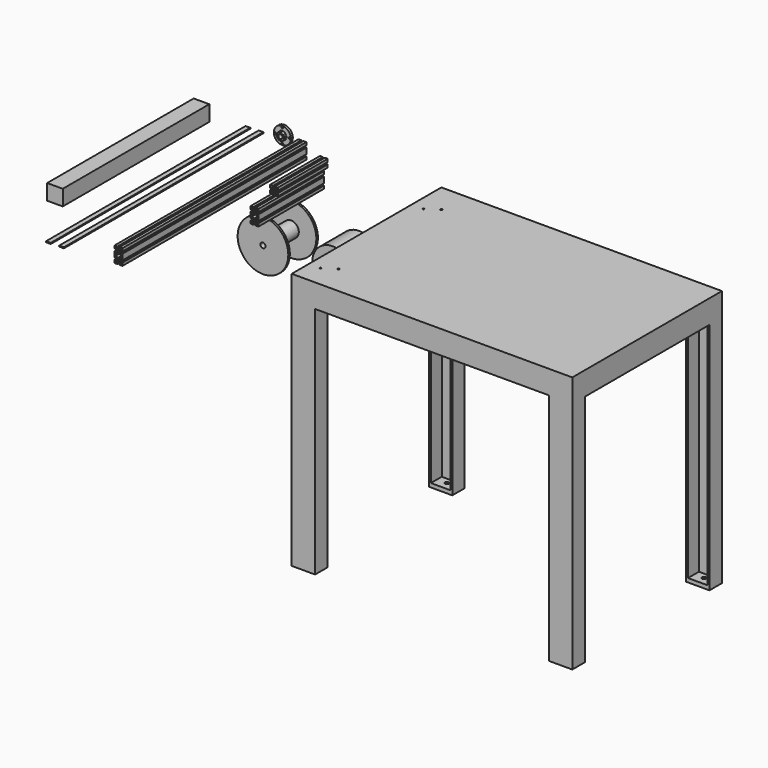
from build123d import *

# Parameters (mm, degrees)
F0_R      = 2.6035
F1_DEPTH  = 749.3
F2_R      = 2.6035
F3_DEPTH  = 203.2
F4_R      = 27.78125
F5_DEPTH  = 7.9375
F6_R      = 12.7
F6_R_2    = 6.858
F7_DEPTH  = 7.9375
F8_R      = 1.27
F10_DEPTH = 76.2
F12_DEPTH = 762
F13_R     = 82.55
F13_R_2   = 8.255
F14_DEPTH = 6.35
F15_R     = 25.4
F15_R_2   = 8.255
F16_DEPTH = 107.95
F17_R     = 82.55
F17_R_2   = 25.4
F17_R_3   = 8.255
F18_DEPTH = 6.35
F19_R     = 66.675
F19_R_2   = 8.255
F20_DEPTH = 107.95
F21_R     = 2.6035
F22_DEPTH = 266.7
F23_W     = 15.24
F23_H     = 3.175
F24_DEPTH = 812.8
F25_W     = 15.24
F25_H     = 3.175
F26_DEPTH = 812.8
F28_DEPTH = 12.7
F30_DEPTH = 12.7
F32_DEPTH = 12.7
F34_DEPTH = 12.7
F35_W     = 50.8
F35_H     = 596.9
F36_DEPTH = 50.8


with BuildPart() as f1:
    # F0 (on Front) → F1 (new body)
    with BuildSketch(Plane.XZ):
        Polygon((-3.2385, 4.5085), (-4.5085, 4.5085), (-4.5085, 3.2385), (-4.5085, -3.2385), (-4.5085, -4.5085), (-3.2385, -4.5085), (3.2385, -4.5085), (4.5085, -4.5085), (4.5085, -3.2385), (4.5085, 3.2385), (4.5085, 4.5085), (3.2385, 4.5085), align=None)
        Circle(F0_R, mode=Mode.SUBTRACT)
        Polygon((-4.5085, -4.5085), (-4.5085, -3.2385), (-10.4902, -7.4295), (-10.4902, -3.2385), (-12.7, -3.2385), (-12.7, -12.7), (-3.2385, -12.7), (-3.2385, -10.4902), (-7.4295, -10.4902), (-3.2385, -4.5085), align=None)
        Polygon((10.4902, -7.4295), (4.5085, -3.2385), (4.5085, -4.5085), (3.2385, -4.5085), (7.4295, -10.4902), (3.2385, -10.4902), (3.2385, -12.7), (12.7, -12.7), (12.7, -3.2385), (10.4902, -3.2385), align=None)
        Polygon((-4.5085, 3.2385), (-4.5085, 4.5085), (-3.2385, 4.5085), (-7.4295, 10.4902), (-7.432806, 12.7), (-12.7, 12.7), (-12.7, 3.2385), (-10.4902, 3.2385), (-10.4902, 7.4295), align=None)
        Polygon((-12.7, 12.7), (-7.432806, 12.7), (-7.436155, 14.938361), (-3.265166, 20.8915), (-4.5085, 20.8915), (-4.5085, 22.1615), (-10.4902, 17.999061), (-10.4902, 22.1615), (-12.7, 22.1615), align=None)
        Polygon((7.4295, 10.4902), (3.2385, 4.5085), (4.5085, 4.5085), (4.5085, 3.2385), (10.4902, 7.4295), (10.4902, 3.2385), (12.7, 3.2385), (12.7, 12.7), (7.426194, 12.7), align=None)
        Polygon((-12.7, 38.1), (-12.7, 28.6385), (-10.4902, 28.6385), (-10.4902, 32.858061), (-4.5085, 28.6385), (-4.5085, 29.9085), (-3.2385, 29.9085), (-7.436155, 35.8902), (-3.2385, 35.8902), (-3.2385, 38.1), align=None)
        Polygon((-4.5085, 20.8915), (-3.265166, 20.8915), (3.251856, 20.8915), (4.5085, 20.8915), (4.5085, 22.1615), (4.5085, 28.6385), (4.5085, 29.9085), (3.2385, 29.9085), (0, 29.9085), (-3.2385, 29.9085), (-4.5085, 29.9085), (-4.5085, 28.6385), (-4.5085, 22.1615), align=None)
        with BuildLine():
            ThreePointArc((2.6035, 25.4), (-1.840953, 23.559047), (0, 28.0035))
            ThreePointArc((0, 28.0035), (1.840953, 27.240953), (2.6035, 25.4))
        make_face(mode=Mode.SUBTRACT)
        Polygon((10.4902, 28.6385), (12.7, 28.6385), (12.7, 38.1), (3.2385, 38.1), (3.2385, 35.8902), (7.422845, 35.8902), (3.2385, 29.9085), (4.5085, 29.9085), (4.5085, 28.6385), (10.4902, 32.858061), align=None)
        Polygon((7.422845, 14.938361), (7.426194, 12.7), (12.7, 12.7), (12.7, 22.1615), (10.4902, 22.1615), (10.4902, 17.999061), (4.5085, 22.1615), (4.5085, 20.8915), (3.251856, 20.8915), align=None)
    extrude(amount=F1_DEPTH)


with BuildPart() as f3:
    # F2 (on Front) → F3 (new body)
    with BuildSketch(Plane.XZ):
        Polygon((65.21165, -4.37637), (65.21165, -3.10637), (59.22995, -7.29737), (59.22995, -3.10637), (57.02015, -3.10637), (57.02015, -12.56787), (66.48165, -12.56787), (66.48165, -10.35807), (62.29065, -10.35807), (66.48165, -4.37637), align=None)
        Polygon((65.21165, 3.37063), (65.21165, 4.64063), (66.48165, 4.64063), (62.29065, 10.62233), (66.48165, 10.62233), (66.48165, 12.83213), (57.02015, 12.83213), (57.02015, 3.37063), (59.22995, 3.37063), (59.22995, 7.56163), align=None)
        Polygon((77.14965, 10.62233), (72.95865, 4.64063), (74.22865, 4.64063), (74.22865, 3.37063), (80.21035, 7.56163), (80.21035, 4.291052), (80.21035, 3.37063), (82.42015, 3.37063), (82.42015, 12.83213), (72.95865, 12.83213), (72.95865, 10.62233), align=None)
        Polygon((80.21035, -7.29737), (74.22865, -3.10637), (74.22865, -4.37637), (72.95865, -4.37637), (77.14965, -10.35807), (72.95865, -10.35807), (72.95865, -12.56787), (82.42015, -12.56787), (82.42015, -3.10637), (80.21035, -3.10637), align=None)
        Polygon((66.48165, 4.64063), (65.21165, 4.64063), (65.21165, 3.37063), (65.21165, -3.10637), (65.21165, -4.37637), (66.48165, -4.37637), (72.95865, -4.37637), (74.22865, -4.37637), (74.22865, -3.10637), (74.22865, 3.37063), (74.22865, 4.64063), (72.95865, 4.64063), align=None)
        with Locations((69.72015, 0.13213)):
            Circle(F2_R, mode=Mode.SUBTRACT)
    extrude(amount=F3_DEPTH)


with BuildPart() as f5:
    # F4 (on Front) → F5 (new body)
    with BuildSketch(Plane.XZ):
        with Locations((-59.230567, 36.74075)):
            Circle(F4_R)
        with BuildLine():
            ThreePointArc((-56.062631, 60.341583), (-42.392587, 53.57873), (-35.629734, 39.908687))
            ThreePointArc((-35.629734, 39.908687), (-33.249129, 39.059442), (-32.243067, 36.74075))
            ThreePointArc((-32.243067, 36.74075), (-33.249129, 34.422058), (-35.629734, 33.572813))
            ThreePointArc((-35.629734, 33.572813), (-42.392587, 19.90277), (-56.062631, 13.139917))
            ThreePointArc((-56.062631, 13.139917), (-56.057333, 13.034142), (-56.055567, 12.92825))
            ThreePointArc((-56.055567, 12.92825), (-59.336459, 9.755016), (-62.398504, 13.139917))
            ThreePointArc((-62.398504, 13.139917), (-76.068547, 19.90277), (-82.8314, 33.572813))
            ThreePointArc((-82.8314, 33.572813), (-86.218067, 36.74075), (-82.8314, 39.908687))
            ThreePointArc((-82.8314, 39.908687), (-76.068547, 53.57873), (-62.398504, 60.341583))
            ThreePointArc((-62.398504, 60.341583), (-59.336459, 63.726484), (-56.055567, 60.55325))
            ThreePointArc((-56.055567, 60.55325), (-56.057333, 60.447358), (-56.062631, 60.341583))
        make_face(mode=Mode.SUBTRACT)
        with BuildLine():
            Line((-59.230567, 43.59875), (-59.230567, 57.37825))
            ThreePointArc((-59.230567, 57.37825), (-61.399505, 58.234558), (-62.398504, 60.341583))
            ThreePointArc((-62.398504, 60.341583), (-76.068547, 53.57873), (-82.8314, 39.908687))
            ThreePointArc((-82.8314, 39.908687), (-80.724375, 38.909688), (-79.868067, 36.74075))
            Line((-79.868067, 36.74075), (-66.088567, 36.74075))
            ThreePointArc((-66.088567, 36.74075), (-64.079905, 41.590088), (-59.230567, 43.59875))
        make_face()
        with BuildLine():
            ThreePointArc((-35.629734, 33.572813), (-38.593067, 36.74075), (-35.629734, 39.908687))
            ThreePointArc((-35.629734, 39.908687), (-42.392587, 53.57873), (-56.062631, 60.341583))
            ThreePointArc((-56.062631, 60.341583), (-57.061629, 58.234558), (-59.230567, 57.37825))
            Line((-59.230567, 57.37825), (-59.230567, 43.59875))
            ThreePointArc((-59.230567, 43.59875), (-54.381229, 41.590088), (-52.372567, 36.74075))
            ThreePointArc((-52.372567, 36.74075), (-59.230567, 29.88275), (-66.088567, 36.74075))
            Line((-66.088567, 36.74075), (-79.868067, 36.74075))
            ThreePointArc((-79.868067, 36.74075), (-80.724375, 34.571812), (-82.8314, 33.572813))
            ThreePointArc((-82.8314, 33.572813), (-76.068547, 19.90277), (-62.398504, 13.139917))
            ThreePointArc((-62.398504, 13.139917), (-59.230567, 16.10325), (-56.062631, 13.139917))
            ThreePointArc((-56.062631, 13.139917), (-42.392587, 19.90277), (-35.629734, 33.572813))
        make_face()
    extrude(amount=F5_DEPTH)

    # F6 (on face) → F7 (join)
    with BuildSketch(Plane.XZ.offset(7.9375)):
        with Locations((-59.230567, 36.74075)):
            Circle(F6_R)
        with Locations((-59.230567, 36.74075)):
            Circle(F6_R_2, mode=Mode.SUBTRACT)
    extrude(amount=F7_DEPTH)

    # F8
    f8_edges = [f5.edges().sort_by_distance(p)[0] for p in [
        (-71.930567, -15.875, 36.74075),
        (-71.930567, -7.9375, 36.74075),
    ]]
    fillet(f8_edges, radius=F8_R)


with BuildPart() as f10:
    # F9 (on Top) → F10 (new body)
    with BuildSketch(Plane.XY):
        Polygon((520.913526, -37.587471), (482.813526, -37.587471), (482.813526, -647.187471), (1397.213526, -647.187471), (1397.213526, -37.587471), (559.013526, -37.587471), align=None)
        with BuildLine():
            ThreePointArc((520.913526, -580.115596), (518.135401, -577.337471), (520.913526, -574.559346))
            ThreePointArc((520.913526, -574.559346), (522.877957, -575.37304), (523.691651, -577.337471))
            ThreePointArc((523.691651, -577.337471), (522.877957, -579.301902), (520.913526, -580.115596))
        make_face(mode=Mode.SUBTRACT)
        with BuildLine():
            ThreePointArc((559.013526, -555.112471), (555.838526, -551.937471), (559.013526, -548.762471))
            ThreePointArc((559.013526, -548.762471), (561.25859, -549.692407), (562.188526, -551.937471))
            ThreePointArc((562.188526, -551.937471), (561.25859, -554.182535), (559.013526, -555.112471))
        make_face(mode=Mode.SUBTRACT)
        with BuildLine():
            ThreePointArc((520.913526, -161.015596), (518.135401, -158.237471), (520.913526, -155.459346))
            ThreePointArc((520.913526, -155.459346), (522.877957, -156.27304), (523.691651, -158.237471))
            ThreePointArc((523.691651, -158.237471), (522.877957, -160.201902), (520.913526, -161.015596))
        make_face(mode=Mode.SUBTRACT)
        with BuildLine():
            ThreePointArc((559.013526, -136.012471), (555.838526, -132.837471), (559.013526, -129.662471))
            ThreePointArc((559.013526, -129.662471), (561.25859, -130.592407), (562.188526, -132.837471))
            ThreePointArc((562.188526, -132.837471), (561.25859, -135.082535), (559.013526, -136.012471))
        make_face(mode=Mode.SUBTRACT)
    extrude(amount=F10_DEPTH)

    # F11 (on face) → F12 (join)
    with BuildSketch(Plane(origin=(0, 0, 0), x_dir=(1, 0, 0), z_dir=(0, 0, -1))):
        Polygon((559.013526, 647.187471), (482.813526, 647.187471), (482.813526, 596.387471), (489.163518, 596.387471), (489.163518, 640.83748), (552.663534, 640.83748), (552.663534, 596.387471), (559.013526, 596.387471), align=None)
        Polygon((489.163526, 88.387471), (482.813526, 88.387471), (482.813526, 37.587471), (559.013526, 37.587471), (559.013526, 88.387471), (552.663526, 88.387471), (552.663526, 43.937471), (489.163526, 43.937471), align=None)
        Polygon((1397.213526, 647.187471), (1321.013526, 647.187471), (1321.013526, 596.387471), (1327.363558, 596.387471), (1327.363558, 640.837439), (1390.863494, 640.837439), (1390.863494, 596.387471), (1397.213526, 596.387471), align=None)
        Polygon((1397.213526, 37.587471), (1397.213526, 88.387471), (1390.863526, 88.387471), (1390.863526, 43.937471), (1327.363526, 43.937471), (1327.363526, 88.387471), (1321.013526, 88.387471), (1321.013526, 37.587471), align=None)
    extrude(amount=F12_DEPTH)

    # F27 (on face) → F28 (join)
    with BuildSketch(Plane(origin=(0, 0, -762), x_dir=(1, 0, 0), z_dir=(0, 0, -1))):
        with BuildLine():
            Line((549.488538, 640.83748), (492.338514, 640.83748))
            Line((492.338514, 640.83748), (515.630007, 625.309818))
            ThreePointArc((515.630007, 625.309818), (520.913526, 628.137471), (526.197046, 625.309818))
            Line((526.197046, 625.309818), (549.488538, 640.83748))
        make_face()
        with BuildLine():
            Line((515.630007, 625.309818), (492.338514, 640.83748))
            Line((492.338514, 640.83748), (489.163518, 640.83748))
            Line((489.163518, 640.83748), (489.163518, 600.620799))
            Line((489.163518, 600.620799), (515.630007, 618.265125))
            ThreePointArc((515.630007, 618.265125), (514.563526, 621.787471), (515.630007, 625.309818))
        make_face()
        with BuildLine():
            Line((489.163518, 600.620799), (489.163518, 596.387471))
            Line((489.163518, 596.387471), (552.663534, 596.387471))
            Line((552.663534, 596.387471), (552.663534, 600.620799))
            Line((552.663534, 600.620799), (526.197046, 618.265125))
            ThreePointArc((526.197046, 618.265125), (520.913526, 615.437471), (515.630007, 618.265125))
            Line((515.630007, 618.265125), (489.163518, 600.620799))
        make_face()
        with BuildLine():
            Line((552.663534, 640.83748), (549.488538, 640.83748))
            Line((549.488538, 640.83748), (526.197046, 625.309818))
            ThreePointArc((526.197046, 625.309818), (526.991061, 623.627601), (527.263526, 621.787471))
            ThreePointArc((527.263526, 621.787471), (526.991061, 619.947342), (526.197046, 618.265125))
            Line((526.197046, 618.265125), (552.663534, 600.620799))
            Line((552.663534, 600.620799), (552.663534, 640.83748))
        make_face()
    extrude(amount=-F28_DEPTH)

    # F29 (on face) → F30 (join)
    with BuildSketch(Plane(origin=(0, 0, -762), x_dir=(1, 0, 0), z_dir=(0, 0, -1))):
        with BuildLine():
            Line((552.663526, 88.387471), (489.163526, 88.387471))
            Line((489.163526, 88.387471), (489.163526, 84.154138))
            Line((489.163526, 84.154138), (515.630007, 66.509818))
            ThreePointArc((515.630007, 66.509818), (520.913526, 69.337471), (526.197046, 66.509818))
            Line((526.197046, 66.509818), (552.663526, 84.154138))
            Line((552.663526, 84.154138), (552.663526, 88.387471))
        make_face()
        with BuildLine():
            Line((515.630007, 66.509818), (489.163526, 84.154138))
            Line((489.163526, 84.154138), (489.163526, 43.937471))
            Line((489.163526, 43.937471), (492.338526, 43.937471))
            Line((492.338526, 43.937471), (515.630007, 59.465125))
            ThreePointArc((515.630007, 59.465125), (514.563526, 62.987471), (515.630007, 66.509818))
        make_face()
        with BuildLine():
            Line((515.630007, 59.465125), (492.338526, 43.937471))
            Line((492.338526, 43.937471), (549.488526, 43.937471))
            Line((549.488526, 43.937471), (526.197046, 59.465125))
            ThreePointArc((526.197046, 59.465125), (520.913526, 56.637471), (515.630007, 59.465125))
        make_face()
        with BuildLine():
            Line((552.663526, 43.937471), (552.663526, 84.154138))
            Line((552.663526, 84.154138), (526.197046, 66.509818))
            ThreePointArc((526.197046, 66.509818), (526.991061, 64.827601), (527.263526, 62.987471))
            ThreePointArc((527.263526, 62.987471), (526.991061, 61.147342), (526.197046, 59.465125))
            Line((526.197046, 59.465125), (549.488526, 43.937471))
            Line((549.488526, 43.937471), (552.663526, 43.937471))
        make_face()
    extrude(amount=-F30_DEPTH)

    # F31 (on face) → F32 (join)
    with BuildSketch(Plane(origin=(0, 0, -762), x_dir=(1, 0, 0), z_dir=(0, 0, -1))):
        with BuildLine():
            Line((1353.830007, 625.309818), (1330.538574, 640.837439))
            Line((1330.538574, 640.837439), (1327.363558, 640.837439))
            Line((1327.363558, 640.837439), (1327.363558, 600.620826))
            Line((1327.363558, 600.620826), (1353.830007, 618.265125))
            ThreePointArc((1353.830007, 618.265125), (1352.763526, 621.787471), (1353.830007, 625.309818))
        make_face()
        with BuildLine():
            Line((1387.688478, 640.837439), (1330.538574, 640.837439))
            Line((1330.538574, 640.837439), (1353.830007, 625.309818))
            ThreePointArc((1353.830007, 625.309818), (1359.113526, 628.137471), (1364.397046, 625.309818))
            Line((1364.397046, 625.309818), (1387.688478, 640.837439))
        make_face()
        with BuildLine():
            Line((1390.863494, 640.837439), (1387.688478, 640.837439))
            Line((1387.688478, 640.837439), (1364.397046, 625.309818))
            ThreePointArc((1364.397046, 625.309818), (1365.191061, 623.627601), (1365.463526, 621.787471))
            ThreePointArc((1365.463526, 621.787471), (1365.191061, 619.947342), (1364.397046, 618.265125))
            Line((1364.397046, 618.265125), (1390.863494, 600.620826))
            Line((1390.863494, 600.620826), (1390.863494, 640.837439))
        make_face()
        with BuildLine():
            Line((1327.363558, 600.620826), (1327.363558, 596.387471))
            Line((1327.363558, 596.387471), (1390.863494, 596.387471))
            Line((1390.863494, 596.387471), (1390.863494, 600.620826))
            Line((1390.863494, 600.620826), (1364.397046, 618.265125))
            ThreePointArc((1364.397046, 618.265125), (1359.113526, 615.437471), (1353.830007, 618.265125))
            Line((1353.830007, 618.265125), (1327.363558, 600.620826))
        make_face()
    extrude(amount=-F32_DEPTH)

    # F33 (on face) → F34 (join)
    with BuildSketch(Plane(origin=(0, 0, -762), x_dir=(1, 0, 0), z_dir=(0, 0, -1))):
        with BuildLine():
            Line((1390.863526, 88.387471), (1327.363526, 88.387471))
            Line((1327.363526, 88.387471), (1327.363526, 84.154138))
            Line((1327.363526, 84.154138), (1353.830007, 66.509818))
            ThreePointArc((1353.830007, 66.509818), (1359.113526, 69.337471), (1364.397046, 66.509818))
            Line((1364.397046, 66.509818), (1390.863526, 84.154138))
            Line((1390.863526, 84.154138), (1390.863526, 88.387471))
        make_face()
        with BuildLine():
            Line((1353.830007, 66.509818), (1327.363526, 84.154138))
            Line((1327.363526, 84.154138), (1327.363526, 43.937471))
            Line((1327.363526, 43.937471), (1330.538526, 43.937471))
            Line((1330.538526, 43.937471), (1353.830007, 59.465125))
            ThreePointArc((1353.830007, 59.465125), (1352.763526, 62.987471), (1353.830007, 66.509818))
        make_face()
        with BuildLine():
            Line((1353.830007, 59.465125), (1330.538526, 43.937471))
            Line((1330.538526, 43.937471), (1387.688526, 43.937471))
            Line((1387.688526, 43.937471), (1364.397046, 59.465125))
            ThreePointArc((1364.397046, 59.465125), (1359.113526, 56.637471), (1353.830007, 59.465125))
        make_face()
        with BuildLine():
            Line((1390.863526, 43.937471), (1390.863526, 84.154138))
            Line((1390.863526, 84.154138), (1364.397046, 66.509818))
            ThreePointArc((1364.397046, 66.509818), (1365.191061, 64.827601), (1365.463526, 62.987471))
            ThreePointArc((1365.463526, 62.987471), (1365.191061, 61.147342), (1364.397046, 59.465125))
            Line((1364.397046, 59.465125), (1387.688526, 43.937471))
            Line((1387.688526, 43.937471), (1390.863526, 43.937471))
        make_face()
    extrude(amount=-F34_DEPTH)


with BuildPart() as f14:
    # F13 (on Front) → F14 (new body)
    with BuildSketch(Plane.XZ):
        with Locations((-32.147106, -223.969892)):
            Circle(F13_R)
        with Locations((-32.147106, -223.969892)):
            Circle(F13_R_2, mode=Mode.SUBTRACT)
    extrude(amount=F14_DEPTH)

    # F15 (on face) → F16 (join)
    with BuildSketch(Plane.XZ.offset(6.35)):
        with Locations((-32.147106, -223.969892)):
            Circle(F15_R)
        with Locations((-32.147106, -223.969892)):
            Circle(F15_R_2, mode=Mode.SUBTRACT)
    extrude(amount=F16_DEPTH)

    # F17 (on face) → F18 (join)
    with BuildSketch(Plane.XZ.offset(114.3)):
        with Locations((-32.147106, -223.969892)):
            Circle(F17_R)
        with Locations((-32.147106, -223.969892)):
            Circle(F17_R_2, mode=Mode.SUBTRACT)
        with Locations((-32.147106, -223.969892)):
            Circle(F17_R_2)
        with Locations((-32.147106, -223.969892)):
            Circle(F17_R_3, mode=Mode.SUBTRACT)
    extrude(amount=F18_DEPTH)


with BuildPart() as f20:
    # F19 (on Front) → F20 (new body)
    with BuildSketch(Plane.XZ):
        with Locations((184.971258, -227.424622)):
            Circle(F19_R)
        with Locations((184.971258, -227.424622)):
            Circle(F19_R_2, mode=Mode.SUBTRACT)
    extrude(amount=F20_DEPTH)


with BuildPart() as f22:
    # F21 (on Front) → F22 (new body)
    with BuildSketch(Plane.XZ):
        Polygon((67.785989, -72.074538), (61.804289, -67.883538), (61.804289, -69.153538), (60.534289, -69.153538), (64.725289, -75.135238), (60.534289, -75.135238), (60.534289, -77.345038), (69.995789, -77.345038), (69.995789, -67.883538), (67.785989, -67.883538), align=None)
        Polygon((52.787289, -69.153538), (52.787289, -67.883538), (46.805589, -72.074538), (46.805589, -67.883538), (44.595789, -67.883538), (44.595789, -77.345038), (54.057289, -77.345038), (54.057289, -75.135238), (49.866289, -75.135238), (54.057289, -69.153538), align=None)
        Polygon((54.057289, -60.136538), (52.787289, -60.136538), (52.787289, -61.406538), (52.787289, -67.883538), (52.787289, -69.153538), (54.057289, -69.153538), (60.534289, -69.153538), (61.804289, -69.153538), (61.804289, -67.883538), (61.804289, -61.406538), (61.804289, -60.136538), (60.534289, -60.136538), align=None)
        with Locations((57.295789, -64.645038)):
            Circle(F21_R, mode=Mode.SUBTRACT)
        Polygon((52.787289, -61.406538), (52.787289, -60.136538), (54.057289, -60.136538), (49.866289, -54.154838), (49.862983, -51.945038), (44.595789, -51.945038), (44.595789, -61.406538), (46.805589, -61.406538), (46.805589, -57.215538), align=None)
        Polygon((64.725289, -54.154838), (60.534289, -60.136538), (61.804289, -60.136538), (61.804289, -61.406538), (67.785989, -57.215538), (67.785989, -61.406538), (69.995789, -61.406538), (69.995789, -51.945038), (64.721983, -51.945038), align=None)
        Polygon((44.595789, -51.945038), (49.862983, -51.945038), (49.859634, -49.706676), (54.030622, -43.753538), (52.787289, -43.753538), (52.787289, -42.483538), (46.805589, -46.645976), (46.805589, -42.483538), (44.595789, -42.483538), align=None)
        Polygon((64.718634, -49.706676), (64.721983, -51.945038), (69.995789, -51.945038), (69.995789, -42.483538), (67.785989, -42.483538), (67.785989, -46.645976), (61.804289, -42.483538), (61.804289, -43.753538), (60.547645, -43.753538), align=None)
        Polygon((44.595789, -26.545038), (44.595789, -36.006538), (46.805589, -36.006538), (46.805589, -31.786976), (52.787289, -36.006538), (52.787289, -34.736538), (54.057289, -34.736538), (49.859634, -28.754838), (54.057289, -28.754838), (54.057289, -26.545038), align=None)
        Polygon((67.785989, -36.006538), (69.995789, -36.006538), (69.995789, -26.545038), (60.534289, -26.545038), (60.534289, -28.754838), (64.718634, -28.754838), (60.534289, -34.736538), (61.804289, -34.736538), (61.804289, -36.006538), (67.785989, -31.786976), align=None)
        Polygon((52.787289, -43.753538), (54.030622, -43.753538), (60.547645, -43.753538), (61.804289, -43.753538), (61.804289, -42.483538), (61.804289, -36.006538), (61.804289, -34.736538), (60.534289, -34.736538), (57.295789, -34.736538), (54.057289, -34.736538), (52.787289, -34.736538), (52.787289, -36.006538), (52.787289, -42.483538), align=None)
        with BuildLine():
            ThreePointArc((59.899289, -39.245038), (55.454836, -41.08599), (57.295789, -36.641538))
            ThreePointArc((57.295789, -36.641538), (59.136741, -37.404085), (59.899289, -39.245038))
        make_face(mode=Mode.SUBTRACT)
    extrude(amount=F22_DEPTH)


with BuildPart() as f24:
    # F23 (on Front) → F24 (new body)
    with BuildSketch(Plane.XZ):
        with Locations((-134.927564, 19.492597)):
            Rectangle(F23_W, F23_H)
    extrude(amount=F24_DEPTH)


with BuildPart() as f26:
    # F25 (on Front) → F26 (new body)
    with BuildSketch(Plane.XZ):
        with Locations((-177.705475, 18.220534)):
            Rectangle(F25_W, F25_H)
    extrude(amount=F26_DEPTH)


with BuildPart() as f36:
    # F35 (on Top) → F36 (new body)
    with BuildSketch(Plane.XY):
        with Locations((-320.786732, -308.855138)):
            Rectangle(F35_W, F35_H)
    extrude(amount=F36_DEPTH)


solid = Compound([f1.part, f3.part, f5.part, f10.part, f14.part, f20.part, f22.part, f24.part, f26.part, f36.part])
